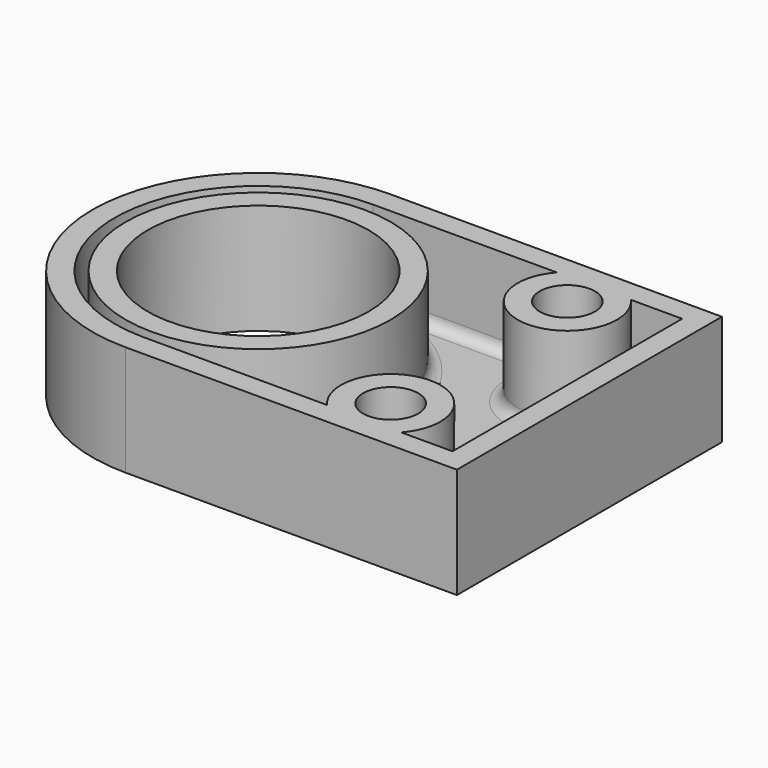
from build123d import *

# Parameters (mm, degrees)
F0_R         = 3.175
F0_R_2       = 12.7
F1_DEPTH     = 12.7
F2_T         = -2.54
F3_T1_DEPTH  = 33.02
F3_T6_DEPTH  = 24.3152905029
F3_S7_R      = 5.715
F3_T8_DEPTH  = 14
F3_T12_ANGLE = 253.7190819507
F3_T17_ANGLE = 73.6440624835
F3_T22_DEPTH = 9.0752905029
F3_S23_R     = 5.715
F3_T24_DEPTH = 6
F3_T28_DEPTH = 9.0752905029
F3_S29_R     = 5.715
F3_T30_DEPTH = 6
F3_T34_ANGLE = 73.6440624835
F3_T39_ANGLE = 253.7190819507
F3_T44_DEPTH = 24.3152905029
F3_S45_R     = 5.715
F3_T46_DEPTH = 14
F3_T48_ANGLE = 180


# Not quite as in the source:
# - a fillet or chamfer that OpenCascade refuses, or shapes differently, is made with other operations: its cross-section is extruded or revolved along the edge and cut away or added


with BuildPart() as f1:
    # F0 (on Top) → F1 (new body)
    with BuildSketch(Plane.XY):
        with BuildLine():
            Line((28.575, -19.05), (28.575, 19.05))
            Line((28.575, 19.05), (-9.525, 19.05))
            ThreePointArc((-9.525, 19.05), (-28.575, 0), (-9.525, -19.05))
            Line((-9.525, -19.05), (28.575, -19.05))
        make_face()
        with Locations((15.875, -12.7)):
            Circle(F0_R, mode=Mode.SUBTRACT)
        with Locations((-9.525, 0)):
            Circle(F0_R_2, mode=Mode.SUBTRACT)
        with Locations((15.875, 12.7)):
            Circle(F0_R, mode=Mode.SUBTRACT)
    extrude(amount=F1_DEPTH)

    # F2
    f2_openings = [f1.faces().sort_by_distance(p)[0] for p in [
        (5.241716, 0, 12.7),
    ]]
    offset(amount=F2_T, openings=f2_openings)

    # F3: fillet of radius 1.27 on 11 edges, made by hand

    # F3_s2 → F3_t1 (join)
    with BuildSketch(Plane.XZ.offset(-16.51)):
        with BuildLine():
            ThreePointArc((26.035, 3.81), (25.6630256121, 2.9119743879), (24.765, 2.54))
            Line((24.765, 2.54), (26.035, 2.54))
            Line((26.035, 2.54), (26.035, 3.81))
        make_face()
    extrude(amount=F3_T1_DEPTH)


with BuildPart() as f3_tool4:
    # F3_s5 → F3_t6 (new body)
    with BuildSketch(Plane.YZ.offset(-9.525)):
        with BuildLine():
            ThreePointArc((-16.51, 3.81), (-16.1380256121, 2.9119743879), (-15.24, 2.54))
            Line((-15.24, 2.54), (-16.51, 2.54))
            Line((-16.51, 2.54), (-16.51, 3.81))
        make_face()
    extrude(amount=F3_T6_DEPTH)

    # F3_s7 → F3_t8 (cut, symmetric)
    with BuildSketch(Plane.XY.offset(3.2)):
        with Locations((15.875, -12.7)):
            Circle(F3_S7_R)
    extrude(amount=F3_T8_DEPTH, both=True, mode=Mode.SUBTRACT)


with BuildPart() as f1_1:
    add(f1.part)

    # F3_t3: union F3_tool4
    add(f3_tool4.part)


with BuildPart() as f3_tool10:
    # F3_s11 → F3_t12 (revolve)
    with BuildSketch(Plane(origin=(18.0449433807, -5.2701877221, 0), x_dir=(0, 0, 1), z_dir=(0.9598987128, -0.2803470371, 0))):
        with BuildLine():
            ThreePointArc((3.81, 13.4552044392), (2.9119743879, 13.8271788271), (2.54, 14.7252044392))
            Line((2.54, 14.7252044392), (2.54, 13.4552044392))
            Line((2.54, 13.4552044392), (3.81, 13.4552044392))
        make_face()
    revolve(axis=Axis((15.875, -12.7, 2.54), (0, 0, -1)), revolution_arc=F3_T12_ANGLE)

    split(bisect_by=Plane.XZ.offset(16.51), keep=Keep.BOTTOM)


with BuildPart() as f1_2:
    add(f1_1.part)

    # F3_t9: union F3_tool10
    add(f3_tool10.part)


with BuildPart() as f3_tool15:
    # F3_s16 → F3_t17 (revolve)
    with BuildSketch(Plane.XZ.offset(12.7)):
        with BuildLine():
            ThreePointArc((21.59, 3.81), (21.9619743879, 2.9119743879), (22.86, 2.54))
            Line((22.86, 2.54), (21.59, 2.54))
            Line((21.59, 2.54), (21.59, 3.81))
        make_face()
    revolve(axis=Axis((15.875, -12.7, 2.54), (0, 0, -1)), revolution_arc=F3_T17_ANGLE)

    split(bisect_by=Plane.XZ.offset(16.51), keep=Keep.BOTTOM)


with BuildPart() as f1_3:
    add(f1_2.part)

    # F3_t14: union F3_tool15
    add(f3_tool15.part)


with BuildPart() as f3_tool20:
    # F3_s21 → F3_t22 (new body)
    with BuildSketch(Plane.YZ.offset(16.9597094971)):
        with BuildLine():
            ThreePointArc((-16.51, 3.81), (-16.1380256121, 2.9119743879), (-15.24, 2.54))
            Line((-15.24, 2.54), (-16.51, 2.54))
            Line((-16.51, 2.54), (-16.51, 3.81))
        make_face()
    extrude(amount=F3_T22_DEPTH)

    # F3_s23 → F3_t24 (cut, symmetric)
    with BuildSketch(Plane.XY.offset(3.2)):
        with Locations((15.875, -12.7)):
            Circle(F3_S23_R)
    extrude(amount=F3_T24_DEPTH, both=True, mode=Mode.SUBTRACT)


with BuildPart() as f1_4:
    add(f1_3.part)

    # F3_t19: union F3_tool20
    add(f3_tool20.part)


with BuildPart() as f3_tool26:
    # F3_s27 → F3_t28 (new body)
    with BuildSketch(Plane.YZ.offset(26.035)):
        with BuildLine():
            ThreePointArc((16.51, 3.81), (16.1380256121, 2.9119743879), (15.24, 2.54))
            Line((15.24, 2.54), (16.51, 2.54))
            Line((16.51, 2.54), (16.51, 3.81))
        make_face()
    extrude(amount=-F3_T28_DEPTH)

    # F3_s29 → F3_t30 (cut, symmetric)
    with BuildSketch(Plane.XY.offset(3.2)):
        with Locations((15.875, 12.7)):
            Circle(F3_S29_R)
    extrude(amount=F3_T30_DEPTH, both=True, mode=Mode.SUBTRACT)


with BuildPart() as f1_5:
    add(f1_4.part)

    # F3_t25: union F3_tool26
    add(f3_tool26.part)


with BuildPart() as f3_tool32:
    # F3_s33 → F3_t34 (revolve)
    with BuildSketch(Plane(origin=(11.1844694654, -3.2824241778, 0), x_dir=(0, 0, 1), z_dir=(-0.9595308214, 0.281603627, 0))):
        with BuildLine():
            ThreePointArc((3.81, 22.3714990108), (2.9119743879, 22.7434733987), (2.54, 23.6414990108))
            Line((2.54, 23.6414990108), (2.54, 22.3714990108))
            Line((2.54, 22.3714990108), (3.81, 22.3714990108))
        make_face()
    revolve(axis=Axis((15.875, 12.7, 2.54), (0, 0, -1)), revolution_arc=F3_T34_ANGLE)

    split(bisect_by=Plane.XZ.offset(-16.51), keep=Keep.TOP)


with BuildPart() as f1_6:
    add(f1_5.part)

    # F3_t31: union F3_tool32
    add(f3_tool32.part)


with BuildPart() as f3_tool37:
    # F3_s38 → F3_t39 (revolve)
    with BuildSketch(Plane.XZ.offset(-12.7)):
        with BuildLine():
            ThreePointArc((21.59, 3.81), (21.9619743879, 2.9119743879), (22.86, 2.54))
            Line((22.86, 2.54), (21.59, 2.54))
            Line((21.59, 2.54), (21.59, 3.81))
        make_face()
    revolve(axis=Axis((15.875, 12.7, 2.54), (0, 0, -1)), revolution_arc=F3_T39_ANGLE)

    split(bisect_by=Plane.XZ.offset(-16.51), keep=Keep.TOP)


with BuildPart() as f1_7:
    add(f1_6.part)

    # F3_t36: union F3_tool37
    add(f3_tool37.part)


with BuildPart() as f3_tool42:
    # F3_s43 → F3_t44 (new body)
    with BuildSketch(Plane.YZ.offset(14.7902905029)):
        with BuildLine():
            ThreePointArc((16.51, 3.81), (16.1380256121, 2.9119743879), (15.24, 2.54))
            Line((15.24, 2.54), (16.51, 2.54))
            Line((16.51, 2.54), (16.51, 3.81))
        make_face()
    extrude(amount=-F3_T44_DEPTH)

    # F3_s45 → F3_t46 (cut, symmetric)
    with BuildSketch(Plane.XY.offset(3.2)):
        with Locations((15.875, 12.7)):
            Circle(F3_S45_R)
    extrude(amount=F3_T46_DEPTH, both=True, mode=Mode.SUBTRACT)


with BuildPart() as f1_8:
    add(f1_7.part)

    # F3_t41: union F3_tool42
    add(f3_tool42.part)

    # F3_s47 → F3_t48 (revolve)
    with BuildSketch(Plane.YZ.offset(-9.525)):
        with BuildLine():
            ThreePointArc((-16.51, 3.81), (-16.1380256121, 2.9119743879), (-15.24, 2.54))
            Line((-15.24, 2.54), (-16.51, 2.54))
            Line((-16.51, 2.54), (-16.51, 3.81))
        make_face()
    revolve(axis=Axis((-9.525, 0, 2.54), (0, 0, -1)), revolution_arc=F3_T48_ANGLE)

    # F3_s49 → F3_t50 (revolve)
    with BuildSketch(Plane.XZ):
        with BuildLine():
            ThreePointArc((6.985, 2.54), (6.0869743879, 2.9119743879), (5.715, 3.81))
            Line((5.715, 3.81), (5.715, 2.54))
            Line((5.715, 2.54), (6.985, 2.54))
        make_face()
    revolve(axis=Axis((-9.525, 0, 2.54), (0, 0, -1)))


solid = f1_8.part
